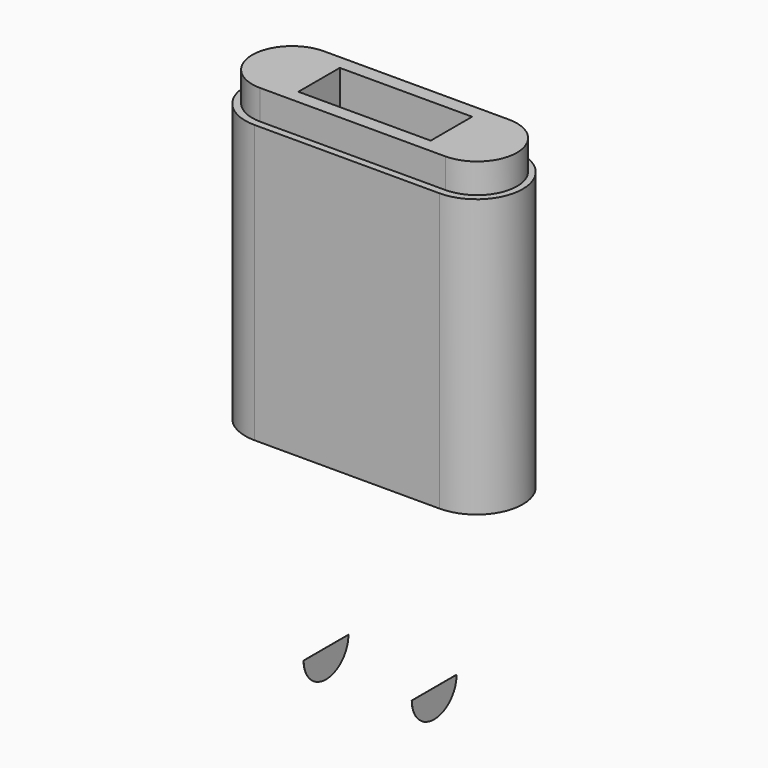
from build123d import *

# Parameters (mm, degrees)
F0_W      = 50.8
F0_H      = 25.4
F1_DEPTH  = 76.2
F2_W      = 50.8
F2_H      = 21.8636197969
F3_DEPTH  = 8.128
F4_W      = 36.3274179399
F4_H      = 14.2120234668
F5_DEPTH  = 25.4
F6_W      = 29.4962525368
F6_H      = 4.1017830372
F7_DEPTH  = 16.002
F11_DEPTH = 0.0254
F13_DEPTH = 0.0254


with BuildPart() as f1:
    # F0 (on Top) → F1 (new body)
    with BuildSketch(Plane.XY):
        with Locations((-4.6053994447, 2.627191287)):
            Rectangle(F0_W, F0_H)
        with BuildLine():
            Line((-30.0053994447, -10.072808713), (-30.0053994447, 15.327191287))
            ThreePointArc((-30.0053994447, 15.327191287), (-42.7053994447, 2.627191287), (-30.0053994447, -10.072808713))
        make_face()
        with BuildLine():
            ThreePointArc((20.7946005553, -10.072808713), (33.4946005553, 2.627191287), (20.7946005553, 15.327191287))
            Line((20.7946005553, 15.327191287), (20.7946005553, -10.072808713))
        make_face()
    extrude(amount=F1_DEPTH)

    # F2 (on face) → F3 (join)
    with BuildSketch(Plane.XY.offset(76.2)):
        with BuildLine():
            ThreePointArc((20.7946005553, -8.0985203385), (31.7264104538, 2.8332895599), (20.7946005553, 13.7650994584))
            Line((20.7946005553, 13.7650994584), (20.7946005553, -8.0985203385))
        make_face()
        with Locations((-4.6053994447, 2.8332895599)):
            Rectangle(F2_W, F2_H)
        with BuildLine():
            Line((-30.0053994447, -8.0985203385), (-30.0053994447, 13.7650994584))
            ThreePointArc((-30.0053994447, 13.7650994584), (-40.9372093432, 2.8332895599), (-30.0053994447, -8.0985203385))
        make_face()
    extrude(amount=F3_DEPTH)

    # F4 (on face) → F5 (cut)
    with BuildSketch(Plane.XY.offset(84.328)):
        with Locations((-4.3616183102, 2.7527492493)):
            Rectangle(F4_W, F4_H)
    extrude(amount=-F5_DEPTH, mode=Mode.SUBTRACT)

    # F6 (on face) → F7 (join)
    with BuildSketch(Plane.XY.offset(58.928)):
        with Locations((-4.9228500575, 5.587247666)):
            Rectangle(F6_W, F6_H)
    extrude(amount=F7_DEPTH)


with BuildPart() as f11:
    # F10 (on face) → F11 (new body)
    with BuildSketch(Plane(origin=(-19.4541122764, 0, 0), x_dir=(0, -1, 0), z_dir=(-1, 0, 0))):
        with BuildLine():
            Line((6.3879964873, -51.308), (-8.9785149321, -51.308))
            ThreePointArc((-8.9785149321, -51.308), (-1.2952592224, -58.9912557097), (6.3879964873, -51.308))
        make_face()
    extrude(amount=F11_DEPTH)


with BuildPart() as f13:
    # F12 (on face) → F13 (new body)
    with BuildSketch(Plane(origin=(10.243313387, 0, 0), x_dir=(0, -1, 0), z_dir=(-1, 0, 0))):
        with BuildLine():
            Line((6.3879964873, -51.308), (-8.9785149321, -51.308))
            ThreePointArc((-8.9785149321, -51.308), (-1.2952592224, -58.9912557097), (6.3879964873, -51.308))
        make_face()
    extrude(amount=F13_DEPTH)


solid = Compound([f1.part, f11.part, f13.part])
